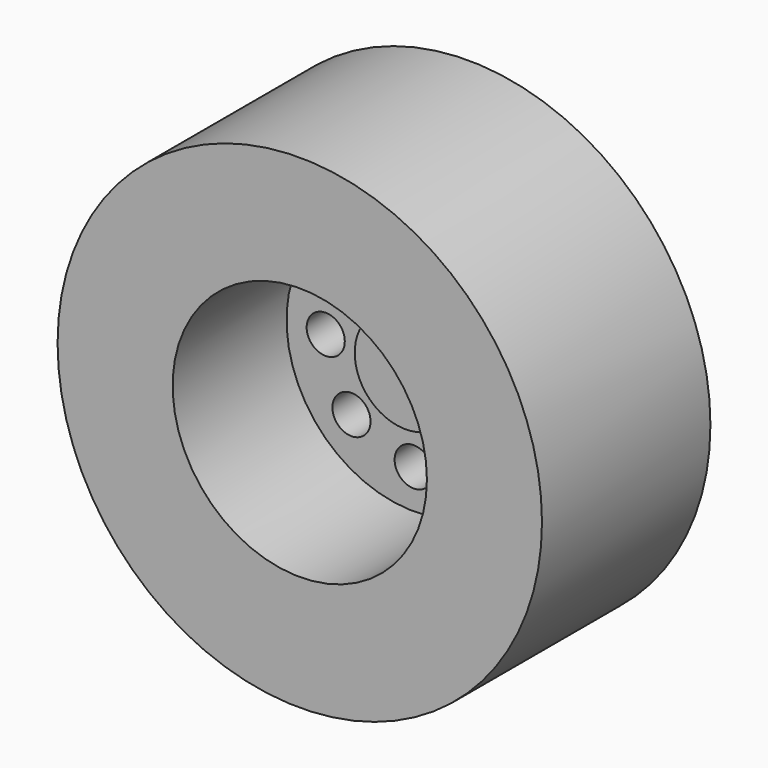
from build123d import *

# Parameters (mm, degrees)
F0_R     = 19.05
F1_DEPTH = 16.5608
F2_R     = 10
F3_DEPTH = 11.2
F4_R     = 4
F5_DEPTH = 0.8
F8_R     = 1.5
F9_DEPTH = 6


# Not quite as in the source:
# - the program builds the solid bodies; features that only make, move or delete a surface that nothing else refers to are left out


with BuildPart() as f1:
    # F0 (on Front) → F1 (new body)
    with BuildSketch(Plane.XZ):
        Circle(F0_R)
    extrude(amount=F1_DEPTH)

    # F2 (on face) → F3 (cut)
    with BuildSketch(Plane.XZ.offset(16.5608)):
        Circle(F2_R)
    extrude(amount=-F3_DEPTH, mode=Mode.SUBTRACT)

    # F4 (on face) → F5 (join)
    with BuildSketch(Plane.XZ.offset(5.3608)):
        Circle(F4_R)
    extrude(amount=F5_DEPTH)

    # F8 (on face) → F9 (cut)
    with BuildSketch(Plane.XZ.offset(5.3608)):
        with Locations((0, 6.9199060356)):
            Circle(F8_R)
        with Locations((-4.8931124829, 4.8931124829)):
            Circle(F8_R)
        with Locations((-6.9199060356, 0)):
            Circle(F8_R)
        with Locations((-4.8931124829, -4.8931124829)):
            Circle(F8_R)
        with Locations((0, -6.9199060356)):
            Circle(F8_R)
        with Locations((4.8931124829, -4.8931124829)):
            Circle(F8_R)
        with Locations((6.9199060356, 0)):
            Circle(F8_R)
        with Locations((4.8931124829, 4.8931124829)):
            Circle(F8_R)
    extrude(amount=-F9_DEPTH, mode=Mode.SUBTRACT)


solid = f1.part
